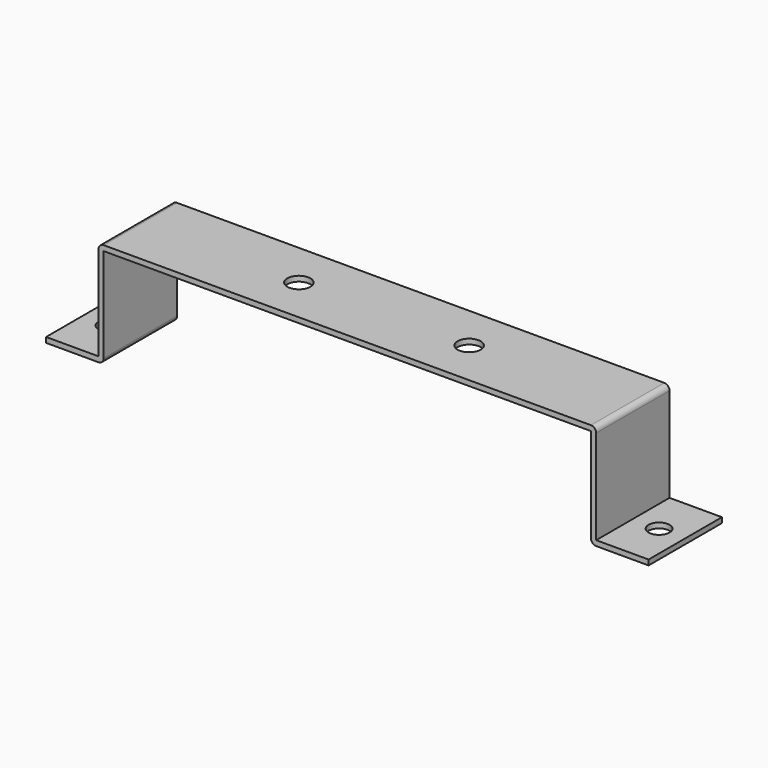
from build123d import *

# Parameters (mm, degrees)
F1_DEPTH = 17.5
F2_R     = 4
F3_DEPTH = 25
F4_R     = 4.4
F5_DEPTH = 25
F6_R     = 2


# Not quite as in the source:
# - a feature names something its author has since deleted; it is built from what else it names


with BuildPart() as f1:
    # F0 (on Front) → F1 (new body, symmetric)
    with BuildSketch(Plane.XZ):
        Polygon((95, -38), (95, 0), (-95, 0), (-95, -38), (-115, -38), (-115, -40), (-93, -40), (-93, -2), (93, -2), (93, -40), (115, -40), (115, -38), align=None)
    extrude(amount=F1_DEPTH, both=True)

    # F2 (on face) → F3 (cut)
    with BuildSketch(Plane.XY.offset(-38)):
        with Locations((-105, 0)):
            Circle(F2_R)
        with Locations((105, 0)):
            Circle(F2_R)
    extrude(amount=-F3_DEPTH, mode=Mode.SUBTRACT)

    # F4 (on face) → F5 (cut)
    with BuildSketch(Plane.XY):
        with Locations((-32.5, 0)):
            Circle(F4_R)
        with Locations((32.5, 0)):
            Circle(F4_R)
    extrude(amount=-F5_DEPTH, mode=Mode.SUBTRACT)

    # F6
    f6_edges = [f1.edges().sort_by_distance(p)[0] for p in [
        (95, 0, 0),
        (-95, 0, 0),
        (-93, 0, -40),
        (93, 0, -40),
    ]]
    fillet(f6_edges, radius=F6_R)


solid = f1.part
